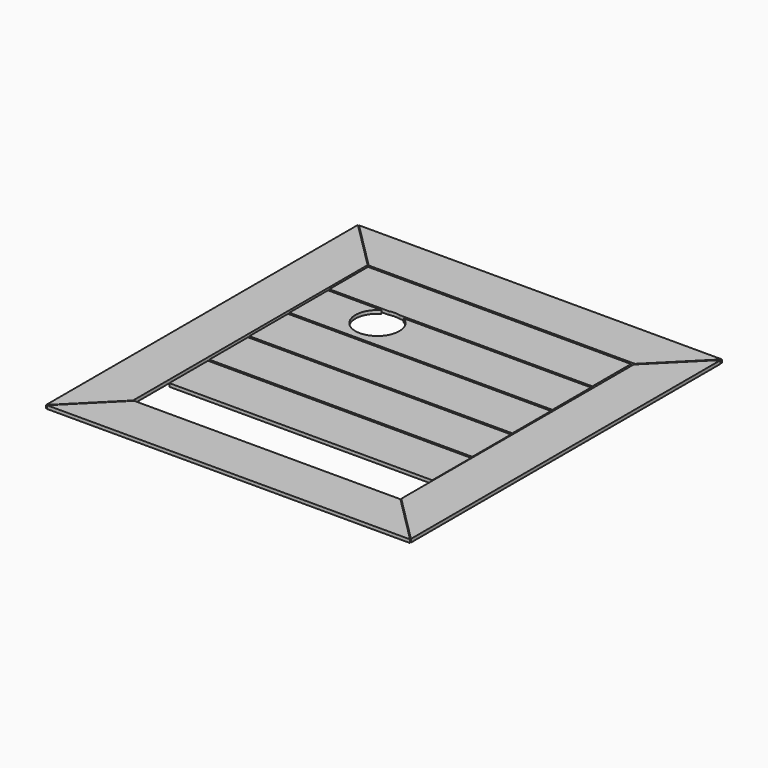
from build123d import *

# Parameters (mm, degrees)
F1_DEPTH      = 19.05
F0_W          = 1520.485255909
F0_H          = 279.4
F2_R          = 127
F3_DEPTH      = 19.051
F3_DEPTH_BACK = 4532


# Not quite as in the source:
# - an extrude ends at something that could not be found from the text; its depth is read off the source's solid


with BuildPart() as f1:
    # F0 (on Top) → F1 (new body)
    with BuildSketch(Plane.XY):
        Polygon((-1552.1603912354, 2430.7818412781), (-1552.1603912354, 176.7163574696), (-1272.7603912354, 456.1163574696), (-1272.7603912354, 2151.3818412781), align=None)
    extrude(amount=F1_DEPTH)


with BuildPart() as f1b:
    # F0 (on Top) → F1, piece 2 (new body)
    with BuildSketch(Plane.XY):
        Polygon((-1545.8103912354, 176.7163574696), (552.5248646736, 176.7163574696), (273.1248646736, 456.1163574696), (-1266.4103912354, 456.1163574696), align=None)
    extrude(amount=F1_DEPTH)


with BuildPart() as f1c:
    # F0 (on Top) → F1, piece 3 (new body)
    with BuildSketch(Plane.XY):
        Polygon((552.5248646736, 2430.7818412781), (-1545.8103912354, 2430.7818412781), (-1266.4103912354, 2151.3818412781), (273.1248646736, 2151.3818412781), align=None)
    extrude(amount=F1_DEPTH)


with BuildPart() as f1d:
    # F0 (on Top) → F1, piece 4 (new body)
    with BuildSketch(Plane.XY):
        Polygon((552.5248646736, 183.0663574696), (552.5248646736, 2421.9541702463), (273.1248646736, 2142.5541702463), (273.1248646736, 462.4663574696), align=None)
    extrude(amount=F1_DEPTH)


with BuildPart() as f1e:
    # F0 (on Top) → F1, piece 5 (new body)
    with BuildSketch(Plane.XY):
        with Locations((-499.8177632809, 1998.9818412781)):
            Rectangle(F0_W, F0_H)
    extrude(amount=F1_DEPTH)


with BuildPart() as f1f:
    # F0 (on Top) → F1, piece 6 (new body)
    with BuildSketch(Plane.XY):
        with Locations((-497.513896589, 1706.8909270095)):
            Rectangle(F0_W, F0_H)
    extrude(amount=F1_DEPTH)


with BuildPart() as f1g:
    # F0 (on Top) → F1, piece 7 (new body)
    with BuildSketch(Plane.XY):
        with Locations((-495.2100298971, 1414.8000127409)):
            Rectangle(F0_W, F0_H)
    extrude(amount=F1_DEPTH)


with BuildPart() as f1h:
    # F0 (on Top) → F1, piece 8 (new body)
    with BuildSketch(Plane.XY):
        with Locations((-492.9061632052, 1122.7090984723)):
            Rectangle(F0_W, F0_H)
    extrude(amount=F1_DEPTH)


with BuildPart() as f1i:
    # F0 (on Top) → F1, piece 9 (new body)
    with BuildSketch(Plane.XY):
        with Locations((-490.6022965133, 830.6181842037)):
            Rectangle(F0_W, F0_H)
    extrude(amount=F1_DEPTH)


with BuildPart() as f3_tool:
    # F2 (on Top) → F3 (new body, two sides)
    with BuildSketch(Plane.XY) as f3_sk:
        with Locations((-884.0888142586, 1736.3681793213)):
            Circle(F2_R)
    extrude(amount=F3_DEPTH)
    extrude(f3_sk.sketch, amount=-F3_DEPTH_BACK)


with BuildPart() as f1e_1:
    add(f1e.part)

    # F3: cut by f3_tool
    add(f3_tool.part, mode=Mode.SUBTRACT)


with BuildPart() as f1f_1:
    add(f1f.part)

    # F3: cut by f3_tool
    add(f3_tool.part, mode=Mode.SUBTRACT)


solid = Compound([f1.part, f1b.part, f1c.part, f1d.part, f1g.part, f1h.part, f1i.part, f1e_1.part, f1f_1.part])
